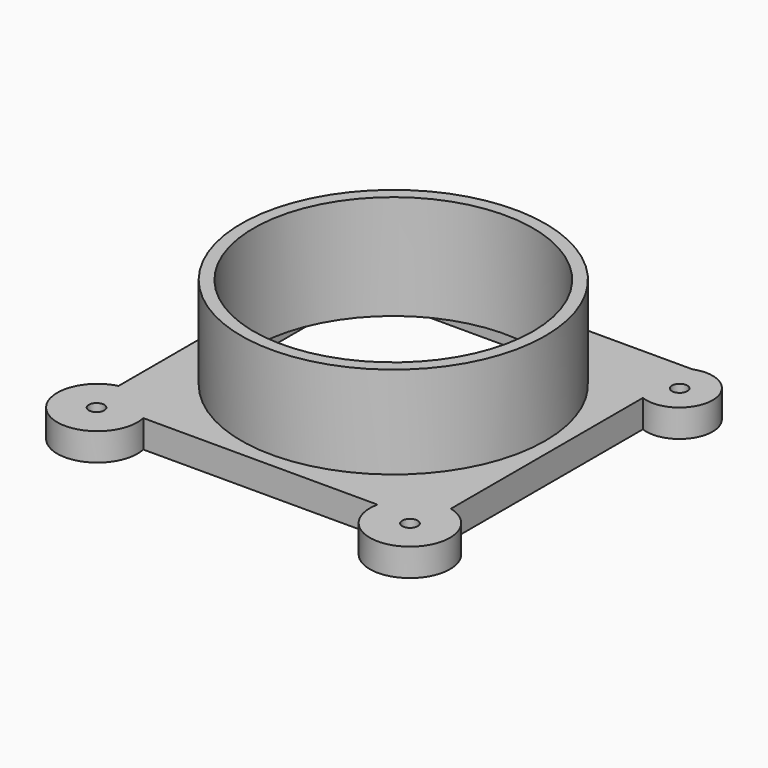
from build123d import *

# Parameters (mm, degrees)
F0_W      = 31.75
F0_H      = 31.75
F1_DEPTH  = 2.54
F2_R      = 28.829
F3_DEPTH  = 25.4
F4_DEPTH  = 2.54
F5_DEPTH  = 2.54
F6_DEPTH  = 2.54
F7_DEPTH  = 2.54
F8_R      = 31.369
F8_R_2    = 28.829
F9_DEPTH  = 19.05
F12_DEPTH = 2.54
F15_DEPTH = 2.54
F17_DEPTH = 3.175
F19_DEPTH = 3.175
F20_R     = 1.5875
F21_DEPTH = 25.4


# Not quite as in the source:
# - a pattern or mirror of a feature is missing from the dataset's text; its kind, count and spacing are read off the source's solid


with BuildPart() as f1:
    # F0 (on Top) → F1 (new body)
    with BuildSketch(Plane.XY):
        with Locations((-15.875, 15.875)):
            Rectangle(F0_W, F0_H)
        with Locations((15.875, -15.875)):
            Rectangle(F0_W, F0_H)
        with Locations((15.875, 15.875)):
            Rectangle(F0_W, F0_H)
        with Locations((-15.875, -15.875)):
            Rectangle(F0_W, F0_H)
    extrude(amount=F1_DEPTH)

    # F2 (on face) → F3 (cut)
    with BuildSketch(Plane.XY.offset(2.54)):
        Circle(F2_R)
    extrude(amount=-F3_DEPTH, mode=Mode.SUBTRACT)

    # F4 (add): a face of the model
    f4_faces = [f1.faces().sort_by_distance(p)[0] for p in [
        (0, -31.75, 1.27),
    ]]
    extrude(f4_faces, amount=F4_DEPTH)

    # F5 (add): a face of the model
    f5_faces = [f1.faces().sort_by_distance(p)[0] for p in [
        (0, 31.75, 1.27),
    ]]
    extrude(f5_faces, amount=F5_DEPTH)

    # F6 (add): a face of the model
    f6_faces = [f1.faces().sort_by_distance(p)[0] for p in [
        (31.75, 0, 1.27),
    ]]
    extrude(f6_faces, amount=F6_DEPTH)

    # F7 (add): a face of the model
    f7_faces = [f1.faces().sort_by_distance(p)[0] for p in [
        (-31.75, 0, 1.27),
    ]]
    extrude(f7_faces, amount=F7_DEPTH)

    # F8 (on face) → F9 (join)
    with BuildSketch(Plane.XY.offset(2.54)):
        Circle(F8_R)
        Circle(F8_R_2, mode=Mode.SUBTRACT)
    extrude(amount=F9_DEPTH)

    # F11 (on face) → F12 (join)
    with BuildSketch(Plane.XY.offset(2.54)):
        with BuildLine():
            Line((34.29, -34.29), (24.1616647691, -34.29))
            ThreePointArc((24.1616647691, -34.29), (36.604718933, -43.052889693), (34.29, -28.0109513551))
            Line((34.29, -28.0109513551), (34.29, -34.29))
        make_face()
    extrude(amount=-F12_DEPTH)

    # F13: F1 across plane


with BuildPart() as f1_1:
    add(f1.part)
    add(f1.part.mirror(Plane(origin=(0, 0, 1.27), x_dir=(0, -1, 0), z_dir=(-1, 0, 0))))

    # F14 (on face) → F15 (join)
    with BuildSketch(Plane.XY.offset(2.54)):
        with BuildLine():
            Line((34.29, 34.29), (34.29, 21.5044934303))
            ThreePointArc((34.29, 21.5044934303), (43.5698705735, 27.8972467151), (34.29, 34.29))
        make_face()
    extrude(amount=-F15_DEPTH)

    # F16: F1 across plane


with BuildPart() as f1_2:
    add(f1_1.part)
    add(f1_1.part.mirror(Plane(origin=(0, 0, 1.27), x_dir=(0, -1, 0), z_dir=(-1, 0, 0))))

    # F17 (add): a face of the model
    f17_faces = [f1_2.faces().sort_by_distance(p)[0] for p in [
        (0, -33.113583232, 0),
    ]]
    extrude(f17_faces, amount=F17_DEPTH)

    # F18 (on face) → F19 (cut)
    with BuildSketch(Plane(origin=(0, 0, -3.175), x_dir=(1, 0, 0), z_dir=(0, 0, -1))):
        with BuildLine():
            Line((0, 30.48), (-27.7283061296, 30.48))
            ThreePointArc((-27.7283061296, 30.48), (-35.4541518447, 42.4181121108), (-30.48, 29.0965121239))
            Line((-30.48, 29.0965121239), (-30.48, 3.2532289624))
            Line((-30.48, 3.2532289624), (-30.48, -27.1199196577))
            ThreePointArc((-30.48, -27.1199196577), (-42.2816797053, -26.6976345281), (-31.094558537, -30.48))
            Line((-31.094558537, -30.48), (0, -30.48))
            Line((0, -30.48), (0, 30.48))
        make_face()
    f19 = extrude(amount=-F19_DEPTH, mode=Mode.SUBTRACT)

    # F19_copies: F19 across plane
    add(f19.mirror(Plane(origin=(0, 0, 0), x_dir=(0, 0, 1), z_dir=(1, 0, 0))), mode=Mode.SUBTRACT)

    # F20 (on face) → F21 (cut)
    with BuildSketch(Plane(origin=(0, 0, 0), x_dir=(1, 0, 0), z_dir=(0, 0, -1))):
        with Locations((-32.3404680081, 36.1273235781)):
            Circle(F20_R)
        with Locations((32.3404680081, 36.1273235781)):
            Circle(F20_R)
        with Locations((36.8319889795, -27.8067924424)):
            Circle(F20_R)
        with Locations((-36.8319889795, -27.8067924424)):
            Circle(F20_R)
    extrude(amount=-F21_DEPTH, mode=Mode.SUBTRACT)


solid = f1_2.part
